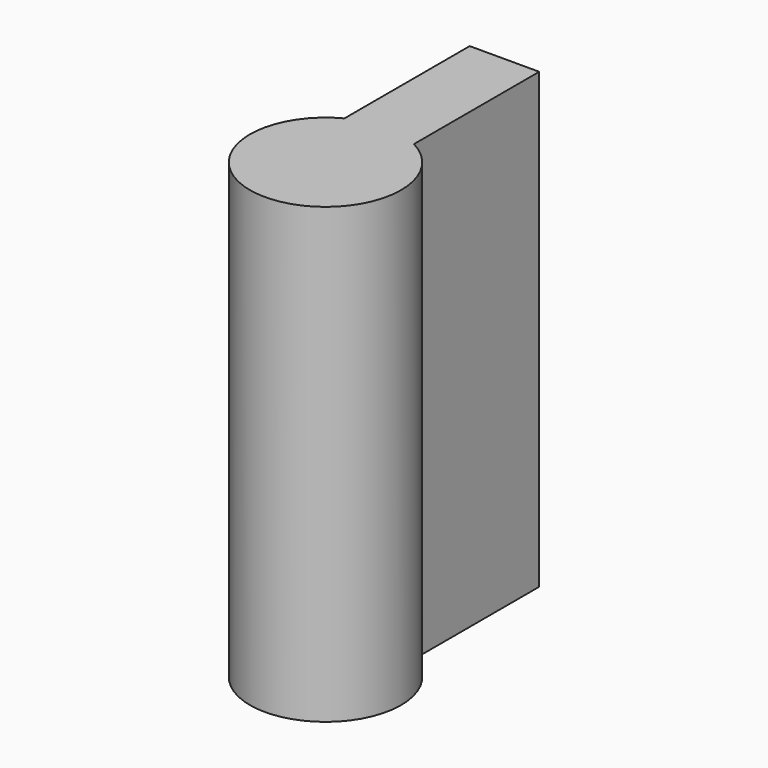
from build123d import *

# Parameters (mm, degrees)
F1_DEPTH = 76.2


with BuildPart() as f1:
    # F0 (on Top) → F1 (new body)
    with BuildSketch(Plane.XY):
        with BuildLine():
            Line((-5.842, 37.592), (-5.842, 11.2765702233))
            ThreePointArc((-5.842, 11.2765702233), (0, -12.7), (5.842, 11.2765702233))
            Line((5.842, 11.2765702233), (5.842, 37.592))
            Line((5.842, 37.592), (-5.842, 37.592))
        make_face()
    extrude(amount=F1_DEPTH)


solid = f1.part
